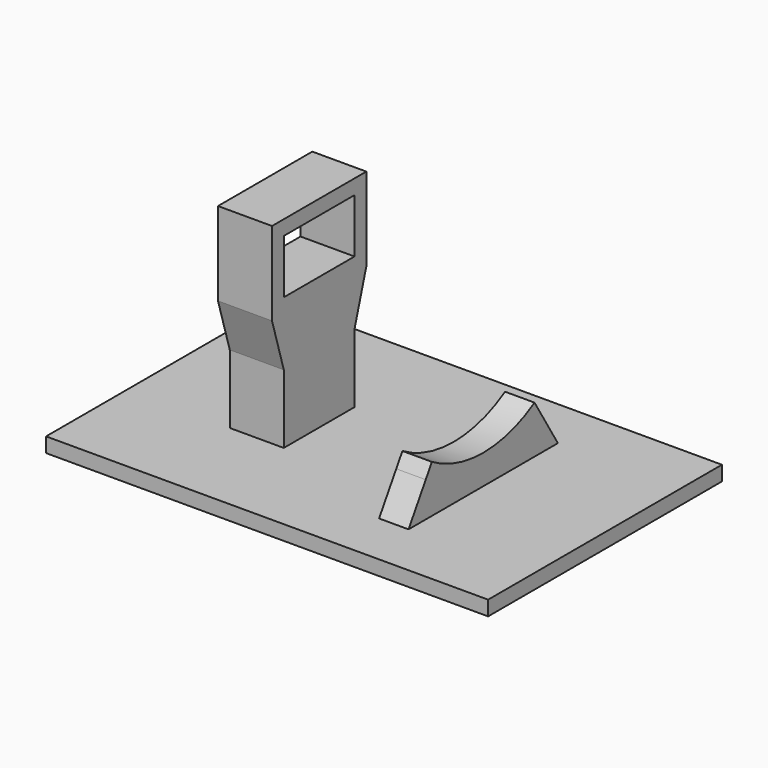
from build123d import *

# Parameters (mm, degrees)
F0_W     = 90
F0_H     = 59.5
F1_DEPTH = 3
F2_W     = 11
F2_H     = 24
F3_DEPTH = 41
F2_W_2   = 6
F2_H_2   = 56
F4_DEPTH = 31
F5_W     = 18
F5_H     = 11
F6_DEPTH = 15
F8_DEPTH = 10


with BuildPart() as f1:
    # F0 (on Top) → F1 (new body)
    with BuildSketch(Plane.XY):
        with Locations((45, 29.3979640784)):
            Rectangle(F0_W, F0_H)
    extrude(amount=F1_DEPTH)

    # F2 (on face) → F3 (join)
    with BuildSketch(Plane.XY.offset(3)):
        with Locations((26.5, 29.1479640784)):
            Rectangle(F2_W, F2_H)
    extrude(amount=F3_DEPTH)

    # F2 (on face) → F4 (join)
    with BuildSketch(Plane.XY.offset(3)):
        with Locations((62, 29.6479640784)):
            Rectangle(F2_W_2, F2_H_2)
    extrude(amount=F4_DEPTH)

    # F5 (on face) → F6 (cut)
    with BuildSketch(Plane(origin=(21, 0, 0), x_dir=(0, -1, 0), z_dir=(-1, 0, 0))):
        Polygon((-41.1479640784, 27), (-41.1479640784, 3), (-38.1479640784, 3), (-38.1479640784, 17), align=None)
        with Locations((-29.1479640784, 35.5)):
            Rectangle(F5_W, F5_H)
        Polygon((-20.1479640784, 17), (-20.1479640784, 3), (-17.1479640784, 3), (-17.1479640784, 27), align=None)
    extrude(amount=-F6_DEPTH, mode=Mode.SUBTRACT)

    # F7 (on face) → F8 (cut)
    with BuildSketch(Plane.YZ.offset(65)):
        with BuildLine():
            Line((29.6479640784, 34), (4.6479640784, 34))
            ThreePointArc((4.6479640784, 34), (7.8351090818, 21.7852811372), (16.5839126302, 12.6849686897))
            Line((16.5839126302, 12.6849686897), (29.6479640784, 34))
        make_face()
        with BuildLine():
            ThreePointArc((16.5839126302, 12.6849686897), (29.6479640784, 9), (42.7120155267, 12.6849686897))
            Line((42.7120155267, 12.6849686897), (29.6479640784, 34))
            Line((29.6479640784, 34), (16.5839126302, 12.6849686897))
        make_face()
        with BuildLine():
            ThreePointArc((42.7120155267, 12.6849686897), (51.460819075, 21.7852811372), (54.6479640784, 34))
            Line((54.6479640784, 34), (29.6479640784, 34))
            Line((29.6479640784, 34), (42.7120155267, 12.6849686897))
        make_face()
        with BuildLine():
            ThreePointArc((16.5839126302, 12.6849686897), (7.8351090818, 21.7852811372), (4.6479640784, 34))
            Line((4.6479640784, 34), (1.6479640784, 34))
            ThreePointArc((1.6479640784, 34), (5.2175664822, 20.3195148737), (15.0162264564, 10.1271649325))
            Line((15.0162264564, 10.1271649325), (16.5839126302, 12.6849686897))
        make_face()
        with BuildLine():
            ThreePointArc((15.0162264564, 10.1271649325), (5.2175664822, 20.3195148737), (1.6479640784, 34))
            Line((1.6479640784, 34), (1.6479640784, 3))
            Line((1.6479640784, 3), (10.6479640784, 3))
            Line((10.6479640784, 3), (15.0162264564, 10.1271649325))
        make_face()
        with BuildLine():
            Line((57.6479640784, 3), (57.6479640784, 34))
            ThreePointArc((57.6479640784, 34), (54.0783616746, 20.3195148737), (44.2797017005, 10.1271649325))
            Line((44.2797017005, 10.1271649325), (48.6479640784, 3))
            Line((48.6479640784, 3), (57.6479640784, 3))
        make_face()
        with BuildLine():
            Line((57.6479640784, 34), (54.6479640784, 34))
            ThreePointArc((54.6479640784, 34), (51.460819075, 21.7852811372), (42.7120155267, 12.6849686897))
            Line((42.7120155267, 12.6849686897), (44.2797017005, 10.1271649325))
            ThreePointArc((44.2797017005, 10.1271649325), (54.0783616746, 20.3195148737), (57.6479640784, 34))
        make_face()
    extrude(amount=-F8_DEPTH, mode=Mode.SUBTRACT)


solid = f1.part
